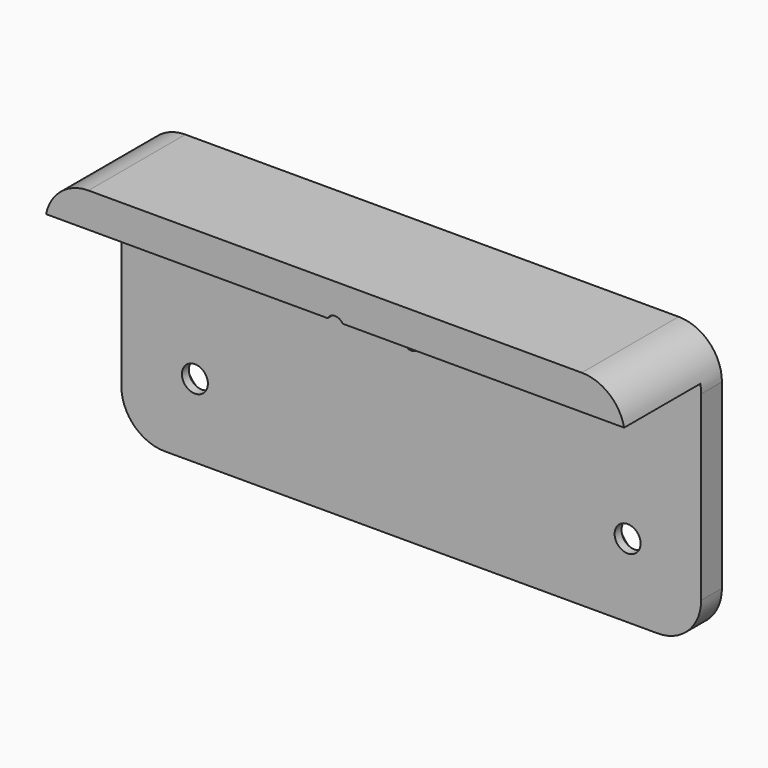
from build123d import *

# Parameters (mm, degrees)
F0_W     = 67
F0_H     = 17
F0_R     = 1.5
F1_DEPTH = 3
F2_DEPTH = 14
F3_R     = 5
F4_R     = 0.99999
F5_SIZE  = 2


# Not quite as in the source:
# - a fillet or chamfer is up to 0.001 mm smaller than in the source, because OpenCascade refuses the exact size


with BuildPart() as f1:
    # F0 (on Front) → F1 (new body)
    with BuildSketch(Plane.XZ):
        Polygon((-33.5, 18.5), (-33.5, 8.5), (33.5, 8.5), (33.5, 18.5), (1, 18.5), (1, 11), (-1, 11), (-1, 18.5), align=None)
        Rectangle(F0_W, F0_H)
        with Locations((-25, 0)):
            Circle(F0_R, mode=Mode.SUBTRACT)
        with Locations((25, 0)):
            Circle(F0_R, mode=Mode.SUBTRACT)
    extrude(amount=F1_DEPTH)

    # F0 (on Front) → F2 (join)
    with BuildSketch(Plane.XZ):
        Polygon((-33.5, 22.5), (-33.5, 18.5), (-1, 18.5), (-1, 19), (1, 19), (1, 18.5), (33.5, 18.5), (33.5, 22.5), align=None)
    extrude(amount=F2_DEPTH)

    # F3
    f3_edges = [f1.edges().sort_by_distance(p)[0] for p in [
        (-33.5, -1.5, -8.5),
        (33.5, -1.5, -8.5),
        (-33.5, -7, 22.5),
        (33.5, -7, 22.5),
    ]]
    fillet(f3_edges, radius=F3_R)

    # F4 (radius 1 in the source; OpenCascade refuses exactly that, so slightly less here)
    f4_edges = [f1.edges().sort_by_distance(p)[0] for p in [
        (-1, -7, 19),
        (1, -7, 19),
        (1, -1.5, 11),
        (-1, -1.5, 11),
    ]]
    fillet(f4_edges, radius=F4_R)

    # F5
    f5_edges = [f1.edges().sort_by_distance(p)[0] for p in [
        (-26.5, 0, 0),
        (23.5, 0, 0),
        (-1, 0, 15),
    ]]
    chamfer(f5_edges, length=F5_SIZE)


solid = f1.part
